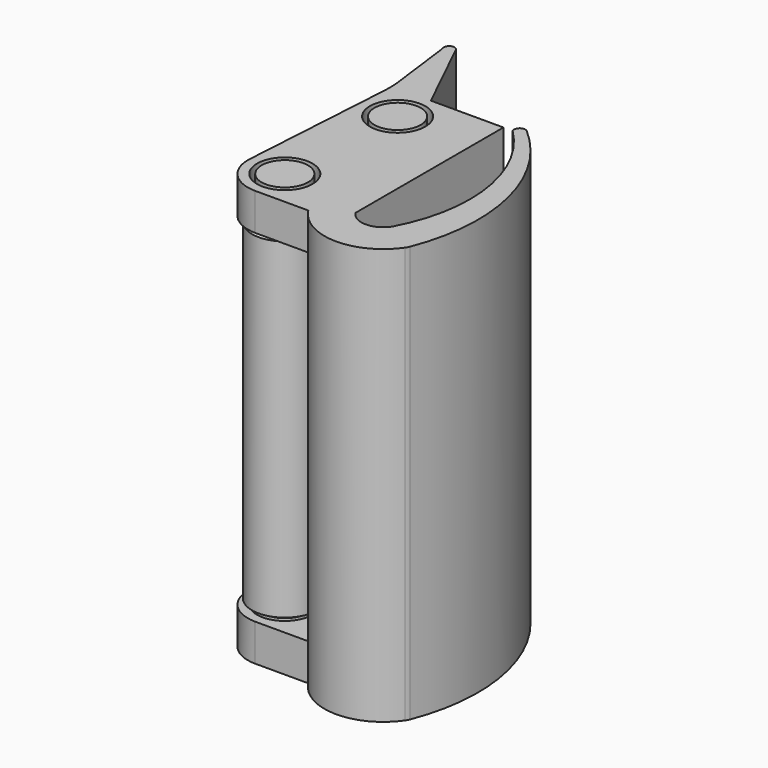
from build123d import *

# Parameters (mm, degrees)
F0_R      = 1.5
F1_DEPTH  = 22.5
F2_W      = 1.5649868256
F2_H      = 18.5
F2_W_2    = 8.4908823588
F2_H_2    = 2
F2_W_3    = 4.0411260356
F3_DEPTH  = 25
F4_DEPTH  = 22.5
F5_DEPTH  = 2
F0_R_2    = 1.25
F5_FACE_R = 1.25
F6_DEPTH  = 0.3
F6_TAPER  = -60
F7_DEPTH  = 17.9
F7_FACE_R = 1.7696152423
F8_DEPTH  = 0.3
F8_TAPER  = 60
F9_DEPTH  = 2
F10_W     = 0.8927135028
F10_H     = 18.5
F11_DEPTH = 25


with BuildPart() as f1:
    # F0 (on Top) → F1 (new body)
    with BuildSketch(Plane.XY):
        with BuildLine():
            Line((-6.2595093475, -0.0628177289), (-5.5704498465, 11.0081995456))
            Line((-5.5704498465, 11.0081995456), (-8.4908092394, 11.0081995456))
            ThreePointArc((-8.4908092394, 11.0081995456), (-9.5714450422, 10.8886817815), (-10.599845389, 10.5359057038))
            Line((-10.599845389, 10.5359057038), (-11.1272968, 2.0614217526))
            ThreePointArc((-11.1272968, 2.0614217526), (-10.5886364868, 0.5675982034), (-9.1311593921, -0.0628177289))
            Line((-9.1311593921, -0.0628177289), (-6.2595093475, -0.0628177289))
        make_face()
        with Locations((-9.1311593921, 1.9371822711)):
            Circle(F0_R, mode=Mode.SUBTRACT)
        with Locations((-8.6910596692, 9.0081995456)):
            Circle(F0_R, mode=Mode.SUBTRACT)
    extrude(amount=F1_DEPTH)

    # F2 (on face) → F3 (cut)
    with BuildSketch(Plane(origin=(-11.2121657678, 0.6978445754, 0), x_dir=(-0.0621197408, -0.998068704, 0), z_dir=(-0.998068704, 0.0621197408, 0))):
        with Locations((-10.6395915159, 11.25)):
            Rectangle(F2_W, F2_H)
        with Locations((-5.6116569237, 11.25)):
            Rectangle(F2_W_2, F2_H)
        with Locations((-5.6116569237, 1)):
            Rectangle(F2_W_2, F2_H_2)
        with Locations((0.6543472735, 11.25)):
            Rectangle(F2_W_3, F2_H)
    extrude(amount=-F3_DEPTH, mode=Mode.SUBTRACT)

    # F0 (on Top) → F4 (join)
    with BuildSketch(Plane.XY):
        with BuildLine():
            ThreePointArc((-10.599845389, 10.5359057038), (-9.5714450422, 10.8886817815), (-8.4908092394, 11.0081995456))
            Line((-8.4908092394, 11.0081995456), (-10.5704498465, 15.2896977961))
            ThreePointArc((-10.5704498465, 15.2896977961), (-10.9289981735, 15.4314206404), (-11.1011234826, 15.0864349228))
            ThreePointArc((-11.1011234826, 15.0864349228), (-11.0828716583, 15.0122379619), (-11.0703382822, 14.9368640104))
            Line((-11.0703382822, 14.9368640104), (-10.6301798393, 11.4776224879))
            ThreePointArc((-10.6301798393, 11.4776224879), (-10.5927809018, 11.0074802207), (-10.599845389, 10.5359057038))
        make_face()
        with BuildLine():
            Line((-4.5704498465, 1.0081995456), (-4.5704498465, 11.0081995456))
            Line((-4.5704498465, 11.0081995456), (-5.5704498465, 11.0081995456))
            Line((-5.5704498465, 11.0081995456), (-6.2595093475, -0.0628177289))
            ThreePointArc((-6.2595093475, -0.0628177289), (-3.6316461386, -1.5412123224), (-0.9489071219, -0.1649031322))
            ThreePointArc((-0.9489071219, -0.1649031322), (-0.8895758539, -0.0673518323), (-0.8417512995, 0.0363268419))
            ThreePointArc((-0.8417512995, 0.0363268419), (-0.4268119196, 6.1501192436), (-3.6132824607, 11.3843372092))
            ThreePointArc((-3.6132824607, 11.3843372092), (-3.9931483806, 11.3801406851), (-4.0704498465, 11.0081995456))
            ThreePointArc((-4.0704498465, 11.0081995456), (-1.6641453193, 6.2566452246), (-2.5704498465, 1.0081995456))
            ThreePointArc((-2.5704498465, 1.0081995456), (-3.5704498465, 0.4581995456), (-4.5704498465, 1.0081995456))
        make_face()
    extrude(amount=F4_DEPTH)

    # F0 (on Top) → F5 (join)
    with BuildSketch(Plane.XY):
        with BuildLine():
            Line((-6.2595093475, -0.0628177289), (-5.5704498465, 11.0081995456))
            Line((-5.5704498465, 11.0081995456), (-8.4908092394, 11.0081995456))
            ThreePointArc((-8.4908092394, 11.0081995456), (-9.5714450422, 10.8886817815), (-10.599845389, 10.5359057038))
            Line((-10.599845389, 10.5359057038), (-11.1272968, 2.0614217526))
            ThreePointArc((-11.1272968, 2.0614217526), (-10.5886364868, 0.5675982034), (-9.1311593921, -0.0628177289))
            Line((-9.1311593921, -0.0628177289), (-6.2595093475, -0.0628177289))
        make_face()
        with Locations((-9.1311593921, 1.9371822711)):
            Circle(F0_R, mode=Mode.SUBTRACT)
        with Locations((-8.6910596692, 9.0081995456)):
            Circle(F0_R, mode=Mode.SUBTRACT)
    extrude(amount=F5_DEPTH)

    # F10 (on face) → F11 (cut)
    with BuildSketch(Plane(origin=(-2.5436906285, -1.235539994, 0), x_dir=(-0.4369134382, 0.8995035561, 0), z_dir=(0.8995035561, 0.4369134382, 0))):
        with Locations((14.0580200475, 11.25)):
            Rectangle(F10_W, F10_H)
    extrude(amount=-F11_DEPTH, mode=Mode.SUBTRACT)


with BuildPart() as f5:
    # F0 (on Top) → F5, piece 2 (new body)
    with BuildSketch(Plane.XY):
        with Locations((-9.1311593921, 1.9371822711)):
            Circle(F0_R_2)
    extrude(amount=F5_DEPTH)

    # F5_face (on face) → F6, piece 2 (join)
    with BuildSketch(Plane(origin=(-8.6910596692, 9.0081995456, 2), x_dir=(1, 0, 0), z_dir=(0, 0, 1))):
        with Locations((-0.4400997229, -7.0710172745)):
            Circle(F5_FACE_R)
    extrude(amount=F6_DEPTH, taper=F6_TAPER)

    # F7#2 (add): a face of the model
    f7_2_faces = [f5.faces().sort_by_distance(p)[0] for p in [
        (-9.1311593921, 1.9371822711, 2.3),
    ]]
    extrude(f7_2_faces, amount=F7_DEPTH)

    # F7_face (on face) → F8, piece 2 (join)
    with BuildSketch(Plane(origin=(-8.6910596692, 9.0081995456, 20.2), x_dir=(1, 0, 0), z_dir=(0, 0, 1))):
        with Locations((-0.4400997229, -7.0710172745)):
            Circle(F7_FACE_R)
    extrude(amount=F8_DEPTH, taper=F8_TAPER)

    # F9#2 (add): a face of the model
    f9_2_faces = [f5.faces().sort_by_distance(p)[0] for p in [
        (-9.1311593921, 1.9371822711, 20.5),
    ]]
    extrude(f9_2_faces, amount=F9_DEPTH)


with BuildPart() as f5b:
    # F0 (on Top) → F5, piece 3 (new body)
    with BuildSketch(Plane.XY):
        with Locations((-8.6910596692, 9.0081995456)):
            Circle(F0_R_2)
    extrude(amount=F5_DEPTH)

    # F5_face (on face) → F6 (join)
    with BuildSketch(Plane(origin=(-8.6910596692, 9.0081995456, 2), x_dir=(1, 0, 0), z_dir=(0, 0, 1))):
        Circle(F5_FACE_R)
    extrude(amount=F6_DEPTH, taper=F6_TAPER)

    # F7 (add): a face of the model
    f7_faces = [f5b.faces().sort_by_distance(p)[0] for p in [
        (-8.6910596692, 9.0081995456, 2.3),
    ]]
    extrude(f7_faces, amount=F7_DEPTH)

    # F7_face (on face) → F8 (join)
    with BuildSketch(Plane(origin=(-8.6910596692, 9.0081995456, 20.2), x_dir=(1, 0, 0), z_dir=(0, 0, 1))):
        Circle(F7_FACE_R)
    extrude(amount=F8_DEPTH, taper=F8_TAPER)

    # F9 (add): a face of the model
    f9_faces = [f5b.faces().sort_by_distance(p)[0] for p in [
        (-8.6910596692, 9.0081995456, 20.5),
    ]]
    extrude(f9_faces, amount=F9_DEPTH)


solid = Compound([f1.part, f5.part, f5b.part])
